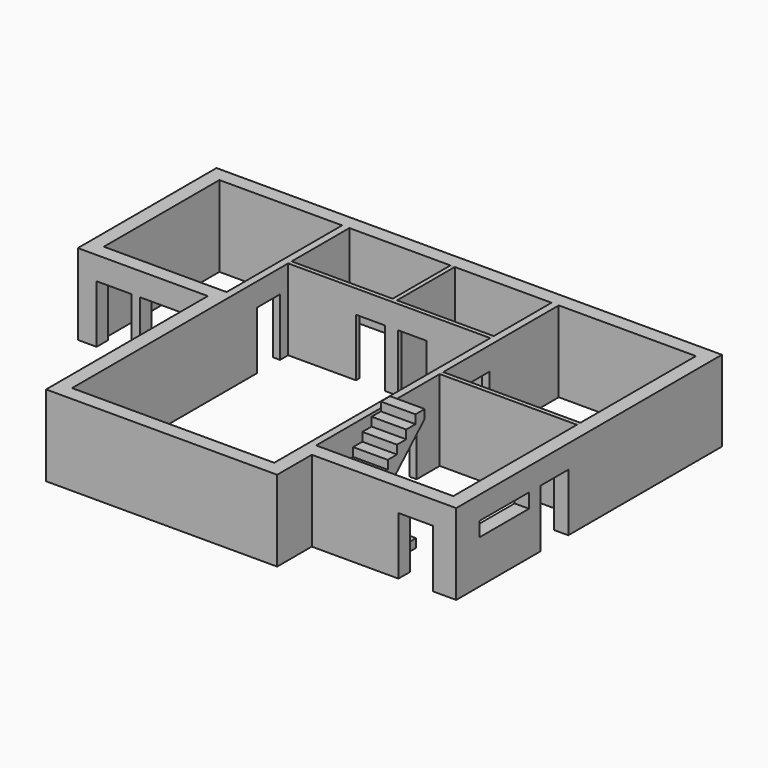
from build123d import *

# Parameters (mm, degrees)
F1_DEPTH  = 2799.9999523163
F3_DEPTH  = 3000
F4_W      = 5000
F4_H      = 2799.9999523163
F5_DEPTH  = 250
F6_W      = 1000
F6_H      = 2000
F7_DEPTH  = 250
F8_W      = 1200
F8_H      = 2000
F9_DEPTH  = 500
F10_W     = 2000
F10_H     = 1200
F11_DEPTH = 500
F12_W     = 10500
F12_H     = 2799.9999523163
F13_DEPTH = 250
F14_W     = 4750
F14_H     = 150
F15_DEPTH = 2800
F16_W     = 1000
F16_H     = 2000
F17_DEPTH = 150
F18_W     = 1000
F18_H     = 2000
F19_DEPTH = 150
F20_W     = 1000
F20_H     = 2000
F21_DEPTH = 250
F22_W     = 1200
F22_H     = 2000
F23_DEPTH = 500
F24_W     = 1200
F24_H     = 2000
F25_DEPTH = 500
F26_W     = 2150
F26_H     = 500
F27_DEPTH = 500
F28_W     = 1200
F28_H     = 2000
F29_DEPTH = 250
F30_W     = 2500
F30_H     = 1200
F31_DEPTH = 1500
F33_DEPTH = 1200
F34_W     = 100
F34_H     = 100
F35_DEPTH = 1400
F36_W     = 1200
F36_H     = 300
F37_DEPTH = 1200
F39_DEPTH = 1200


with BuildPart() as f1:
    # F0 (on Top) → F1 (new body)
    with BuildSketch(Plane.XY):
        Polygon((8875, -3875), (8875, 7625), (-8625, 7625), (-8625, 1625), (-4125, 1625), (-4125, -5375), (3875, -5375), (3875, -3875), align=None)
    extrude(amount=F1_DEPTH)

    # F2 (on Top) → F3 (cut)
    with BuildSketch(Plane.XY):
        Polygon((8375, -3375), (8375, 7125), (-3740.2497768402, 7125), (-8125, 7125), (-8125, 2125), (-3625, 2125), (-3625, -4875), (3375, -4875), (3375, -3375), align=None)
    extrude(amount=F3_DEPTH, mode=Mode.SUBTRACT)

    # F4 (on face) → F5 (join)
    with BuildSketch(Plane.YZ.offset(-3625)):
        with Locations((4625, 1399.9999761581)):
            Rectangle(F4_W, F4_H)
    extrude(amount=-F5_DEPTH)

    # F6 (on face) → F7 (cut, through all)
    with BuildSketch(Plane.YZ.offset(-3625)):
        with Locations((3625, 1000)):
            Rectangle(F6_W, F6_H)
    extrude(amount=-F7_DEPTH, mode=Mode.SUBTRACT)

    # F8 (on face) → F9 (cut, through all)
    with BuildSketch(Plane.XZ.offset(-1625)):
        with Locations((-7375, 1000)):
            Rectangle(F8_W, F8_H)
    extrude(amount=-F9_DEPTH, mode=Mode.SUBTRACT)

    # F10 (on face) → F11 (cut, through all)
    with BuildSketch(Plane.XZ.offset(-1625)):
        with Locations((-5475, 1400)):
            Rectangle(F10_W, F10_H)
    extrude(amount=-F11_DEPTH, mode=Mode.SUBTRACT)

    # F12 (on face) → F13 (join)
    with BuildSketch(Plane(origin=(3375, 0, 0), x_dir=(0, -1, 0), z_dir=(-1, 0, 0))):
        with Locations((-1875, 1399.9999761581)):
            Rectangle(F12_W, F12_H)
    extrude(amount=-F13_DEPTH)

    # F14 (on face) → F15 (join)
    with BuildSketch(Plane.XY):
        Polygon((3375, 4475), (3375, 4625), (25, 4625), (25, 7125), (-125, 7125), (-125, 4625), (-3625, 4625), (-3625, 4475), align=None)
        with Locations((6000, 2050)):
            Rectangle(F14_W, F14_H)
    extrude(amount=F15_DEPTH)

    # F16 (on face) → F17 (cut, through all)
    with BuildSketch(Plane(origin=(0, 4625, 0), x_dir=(-1, 0, 0), z_dir=(0, 1, 0))):
        with Locations((775, 1000)):
            Rectangle(F16_W, F16_H)
    extrude(amount=-F17_DEPTH, mode=Mode.SUBTRACT)

    # F18 (on face) → F19 (cut, through all)
    with BuildSketch(Plane(origin=(0, 4625, 0), x_dir=(-1, 0, 0), z_dir=(0, 1, 0))):
        with Locations((-675, 1000)):
            Rectangle(F18_W, F18_H)
    extrude(amount=-F19_DEPTH, mode=Mode.SUBTRACT)

    # F20 (on face) → F21 (cut, through all)
    with BuildSketch(Plane.YZ.offset(3625)):
        with Locations((3625, 1000)):
            Rectangle(F20_W, F20_H)
    extrude(amount=-F21_DEPTH, mode=Mode.SUBTRACT)

    # F22 (on face) → F23 (cut, through all)
    with BuildSketch(Plane.XZ.offset(3875)):
        with Locations((7475, 1000)):
            Rectangle(F22_W, F22_H)
    extrude(amount=-F23_DEPTH, mode=Mode.SUBTRACT)

    # F24 (on face) → F25 (cut, through all)
    with BuildSketch(Plane.YZ.offset(8875)):
        with Locations((375, 1000)):
            Rectangle(F24_W, F24_H)
    extrude(amount=-F25_DEPTH, mode=Mode.SUBTRACT)

    # F26 (on face) → F27 (cut, through all)
    with BuildSketch(Plane.YZ.offset(8875)):
        with Locations((-1800, 1750)):
            Rectangle(F26_W, F26_H)
    extrude(amount=-F27_DEPTH, mode=Mode.SUBTRACT)

    # F28 (on face) → F29 (cut, through all)
    with BuildSketch(Plane(origin=(3375, 0, 0), x_dir=(0, -1, 0), z_dir=(-1, 0, 0))):
        with Locations((-375, 1000)):
            Rectangle(F28_W, F28_H)
    extrude(amount=-F29_DEPTH, mode=Mode.SUBTRACT)


with BuildPart() as f31:
    # F30 (on face) → F31 (new body)
    with BuildSketch(Plane.XY):
        with Locations((4875, -2775)):
            Rectangle(F30_W, F30_H)
    extrude(amount=F31_DEPTH)

    # F32 (on face) → F33 (cut, through all)
    with BuildSketch(Plane.XZ.offset(3375)):
        Polygon((6125, 300), (6125, 1500), (4825, 1500), (4825, 1200), (5150, 1200), (5150, 900), (5475, 900), (5475, 600), (5800, 600), (5800, 300), align=None)
        Polygon((3625, 1400), (3625, 0), (5800, 0), (4400, 1400), align=None)
    extrude(amount=-F33_DEPTH, mode=Mode.SUBTRACT)

    # F34 (on face) → F35 (join)
    with BuildSketch(Plane(origin=(0, 0, 1400), x_dir=(1, 0, 0), z_dir=(0, 0, -1))):
        with Locations((3675, 3325)):
            Rectangle(F34_W, F34_H)
        with Locations((3675, 2225)):
            Rectangle(F34_W, F34_H)
        with Locations((4350, 2225)):
            Rectangle(F34_W, F34_H)
        with Locations((4350, 3325)):
            Rectangle(F34_W, F34_H)
    extrude(amount=F35_DEPTH)

    # F36 (on face) → F37 (join)
    with BuildSketch(Plane.YZ.offset(4825)):
        with Locations((-2775, 1350)):
            Rectangle(F36_W, F36_H)
        Polygon((-2175, 1500), (-2175, 1200), (-175, 1200), (-175, 3000), (-2175, 3000), align=None)
    extrude(amount=-F37_DEPTH)

    # F38 (on face) → F39 (cut)
    with BuildSketch(Plane.YZ.offset(4825)):
        Polygon((-575, 3000), (-2175, 3000), (-2175, 1800), (-1775, 1800), (-1775, 2100), (-1375, 2100), (-1375, 2400), (-975, 2400), (-975, 2700), (-575, 2700), align=None)
        Polygon((-1775, 1200), (-175, 1200), (-175, 2700), align=None)
    extrude(amount=-F39_DEPTH, mode=Mode.SUBTRACT)


solid = Compound([f1.part, f31.part])
